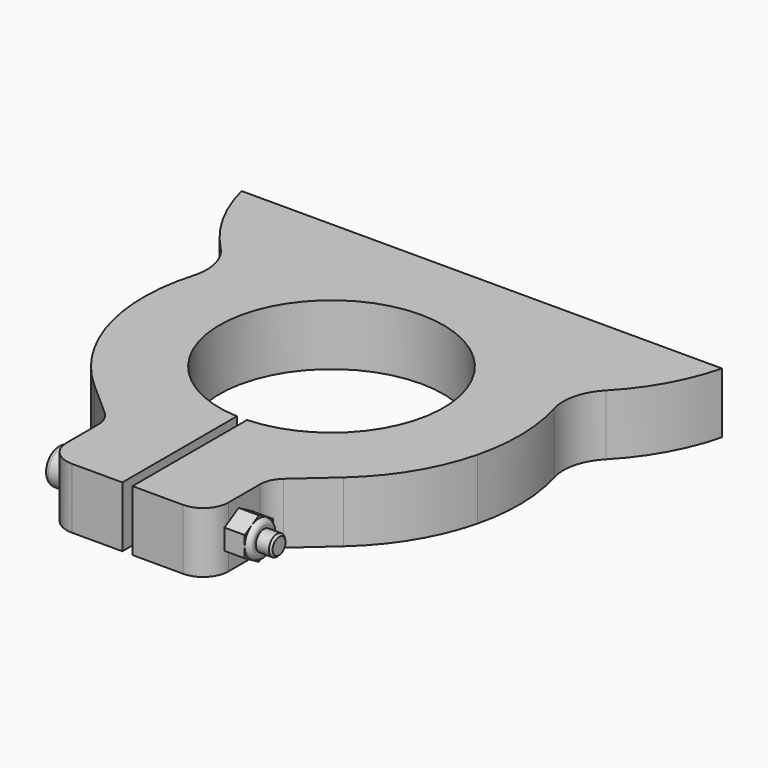
from build123d import *

# Parameters (mm, degrees)
F1_DEPTH  = 12
F2_R      = 37.15
F3_R      = 2
F4_DEPTH  = 63.501
F5_R      = 5
F6_R      = 3.5
F7_DEPTH  = 3.8
F8_R      = 2
F9_DEPTH  = 40
F10_R     = 2
F11_DEPTH = 4
F12_R     = 3.5
F12_R_2   = 2
F13_DEPTH = 1
F14_R     = 0.99999
F15_SIZE  = 0.4
F17_DEPTH = 3
F18_R     = 1
F20_DEPTH = 12.001
F21_R     = 1
F22_DEPTH = 11


# Not quite as in the source:
# - a fillet or chamfer is up to 0.001 mm smaller than in the source, because OpenCascade refuses the exact size


with BuildPart() as f1:
    # F0 (on Top) → F1 (new body)
    with BuildSketch(Plane.XY):
        with BuildLine():
            Line((47.5, 0), (-47.5, 0))
            Line((-47.5, 0), (-33.2750902547, -57.3013205481))
            Line((-33.2750902547, -57.3013205481), (-16, -72.6085300216))
            Line((-16, -72.6085300216), (-16, -87.6085300216))
            Line((-16, -87.6085300216), (-1, -87.6085300216))
            Line((-1, -87.6085300216), (-1, -59.2774151224))
            ThreePointArc((-1, -59.2774151224), (0, -15), (1, -59.2774151224))
            Line((1, -59.2774151224), (1, -87.6085300216))
            Line((1, -87.6085300216), (16, -87.6085300216))
            Line((16, -87.6085300216), (16, -72.6085300216))
            Line((16, -72.6085300216), (33.2750902547, -57.3013205481))
            Line((33.2750902547, -57.3013205481), (47.5, 0))
        make_face()
    extrude(amount=F1_DEPTH)

    # F2
    f2_edges = [f1.edges().sort_by_distance(p)[0] for p in [
        (-33.27509, -57.301321, 6),
        (33.27509, -57.301321, 6),
    ]]
    fillet(f2_edges, radius=F2_R)

    # F3 (on face) → F4 (cut, through all)
    with BuildSketch(Plane(origin=(-16, 0, 0), x_dir=(0, -1, 0), z_dir=(-1, 0, 0))):
        with Locations((80.1085300216, 6)):
            Circle(F3_R)
    extrude(amount=-F4_DEPTH, mode=Mode.SUBTRACT)

    # F5
    f5_edges = [f1.edges().sort_by_distance(p)[0] for p in [
        (-16, -72.60853, 6),
        (-16, -87.60853, 6),
        (16, -87.60853, 6),
        (16, -72.60853, 6),
    ]]
    fillet(f5_edges, radius=F5_R)

    # F19 (on face) → F20 (cut, through all)
    with BuildSketch(Plane.XY.offset(12)):
        with BuildLine():
            ThreePointArc((-38.0832391228, -16.9431848421), (-43.9161727331, -9.0966017337), (-47.5, 0))
            Line((-47.5, 0), (-36.0556124269, -46.1007157545))
            ThreePointArc((-36.0556124269, -46.1007157545), (-37.142105278, -36.3841569879), (-35.6560095209, -26.7206431146))
            ThreePointArc((-35.6560095209, -26.7206431146), (-35.5484448087, -21.5039344632), (-38.0832391228, -16.9431848421))
        make_face()
        with BuildLine():
            ThreePointArc((38.0832391228, -16.9431848421), (35.5484448087, -21.5039344632), (35.6560095209, -26.7206431146))
            ThreePointArc((35.6560095209, -26.7206431146), (37.142105278, -36.3841569879), (36.0556124269, -46.1007157545))
            Line((36.0556124269, -46.1007157545), (47.5, 0))
            ThreePointArc((47.5, 0), (43.9161727331, -9.0966017337), (38.0832391228, -16.9431848421))
        make_face()
    extrude(amount=-F20_DEPTH, mode=Mode.SUBTRACT)

    # F21 (on face) → F22 (cut)
    with BuildSketch(Plane(origin=(0, 0, 0), x_dir=(-1, 0, 0), z_dir=(0, 1, 0))):
        with Locations((-37.5, 6)):
            Circle(F21_R)
        with Locations((-12.5, 6)):
            Circle(F21_R)
        with Locations((12.5, 6)):
            Circle(F21_R)
        with Locations((37.5, 6)):
            Circle(F21_R)
    extrude(amount=-F22_DEPTH, mode=Mode.SUBTRACT)


with BuildPart() as f7:
    # F6 (on face) → F7 (new body)
    with BuildSketch(Plane(origin=(-16, 0, 0), x_dir=(0, -1, 0), z_dir=(-1, 0, 0))):
        with Locations((80.1085300216, 6)):
            Circle(F6_R)
    extrude(amount=F7_DEPTH)

    # F8 (on face) → F9 (join)
    with BuildSketch(Plane.YZ.offset(-16)):
        with Locations((-80.1085300216, 6)):
            Circle(F8_R)
    extrude(amount=F9_DEPTH)

    # F15
    f15_edges = [f7.edges().sort_by_distance(p)[0] for p in [
        (24, -82.10853, 6),
    ]]
    chamfer(f15_edges, length=F15_SIZE)

    # F16 (on face) → F17 (cut)
    with BuildSketch(Plane(origin=(-19.8, 0, 0), x_dir=(0, -1, 0), z_dir=(-1, 0, 0))):
        Polygon((81.1682907283, 3.9481129227), (82.4153967096, 5.8918361553), (81.3556360029, 7.9437232326), (79.0487693149, 8.0518870773), (77.8016633336, 6.1081638447), (78.8614240404, 4.0562767674), align=None)
    extrude(amount=-F17_DEPTH, mode=Mode.SUBTRACT)

    # F18
    f18_edges = [f7.edges().sort_by_distance(p)[0] for p in [
        (-19.8, -76.60853, 6),
    ]]
    fillet(f18_edges, radius=F18_R)


with BuildPart() as f11:
    # F10 (on face) → F11 (new body)
    with BuildSketch(Plane.YZ.offset(16)):
        Polygon((-83.6150630784, 3.9906321255), (-80.1216329251, 1.9585693564), (-76.6150998683, 3.9679372309), (-76.6019969649, 8.0093678745), (-80.0954271181, 10.0414306436), (-83.6019601749, 8.0320627691), align=None)
        with Locations((-80.1085300216, 6)):
            Circle(F10_R, mode=Mode.SUBTRACT)
    extrude(amount=F11_DEPTH)

    # F12 (on face) → F13 (join)
    with BuildSketch(Plane.YZ.offset(20)):
        with Locations((-80.1085300216, 6)):
            Circle(F12_R)
        with Locations((-80.1085300216, 6)):
            Circle(F12_R_2, mode=Mode.SUBTRACT)
    extrude(amount=F13_DEPTH)

    # F14 (radius 1 in the source; OpenCascade refuses exactly that, so slightly less here)
    f14_edges = [f11.edges().sort_by_distance(p)[0] for p in [
        (21, -83.60853, 6),
    ]]
    fillet(f14_edges, radius=F14_R)


solid = Compound([f1.part, f7.part, f11.part])
